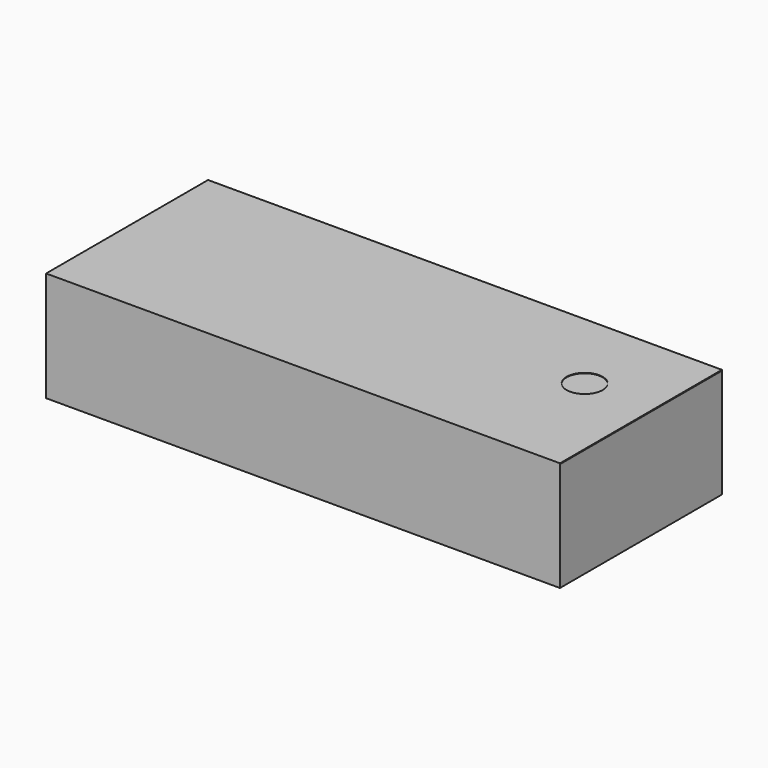
from build123d import *

# Parameters (mm, degrees)
F1_DEPTH = 209.55
F3_DEPTH = 0.4064


# Not quite as in the source:
# - the dataset's text gives a spline's control points without its knots; the knots are read off the source's solid


with BuildPart() as f1:
    # F0 (on Right) → F1 (new body, symmetric)
    with BuildSketch(Plane.YZ):
        Polygon((-165.1, 0), (0, 0), (0, 88.9), (-164.6936, 88.9), (-164.6936, 89.154), (0, 89.154), (0, 89.5604), (-165.1, 89.5604), align=None)
    extrude(amount=F1_DEPTH, both=True)

    # F2 (on face) → F3 (cut, through all)
    with BuildSketch(Plane.XY.offset(89.5604)):
        with BuildLine():
            add(Edge.make_bspline(
                [(163.3854656134, -58.8908826273), (160.6672846134, -56.1726762273), (156.8463118134, -54.5901546273), (153.0019456134, -54.5901546273)],
                knots=[7, 7, 7, 7, 8, 8, 8, 8], degree=3))
            add(Edge.make_bspline(
                [(153.0019456134, -54.5901546273), (149.1579096134, -54.5901546273), (145.3369368134, -56.1726762273), (142.6187304134, -58.8908826273)],
                knots=[0, 0, 0, 0, 1, 1, 1, 1], degree=3))
            add(Edge.make_bspline(
                [(142.6187304134, -58.8908826273), (139.9002446134, -61.6092160273), (138.3175706134, -65.4300110273), (138.3175706134, -69.2745296273), (138.3175706134, -73.1185910273), (139.9002446134, -76.9395384273), (142.6187304134, -79.6580496273)],
                knots=[1, 1, 1, 1, 2, 2, 2, 3, 3, 3, 3], degree=3))
            add(Edge.make_bspline(
                [(142.6187304134, -79.6580496273), (145.3369368134, -82.3760782273), (149.1579096134, -83.9589046273), (153.0019456134, -83.9589046273), (156.8463118134, -83.9589046273), (160.6672846134, -82.3760782273), (163.3854656134, -79.6580496273)],
                knots=[3, 3, 3, 3, 4, 4, 4, 5, 5, 5, 5], degree=3))
            add(Edge.make_bspline(
                [(163.3854656134, -79.6580496273), (166.1039768134, -76.9395384273), (167.6863206134, -73.1185910273), (167.6863206134, -69.2745296273), (167.6863206134, -65.4300110273), (166.1039768134, -61.6092160273), (163.3854656134, -58.8908826273)],
                knots=[5, 5, 5, 5, 6, 6, 6, 7, 7, 7, 7], degree=3))
        make_face()
    extrude(amount=-F3_DEPTH, mode=Mode.SUBTRACT)


solid = f1.part
